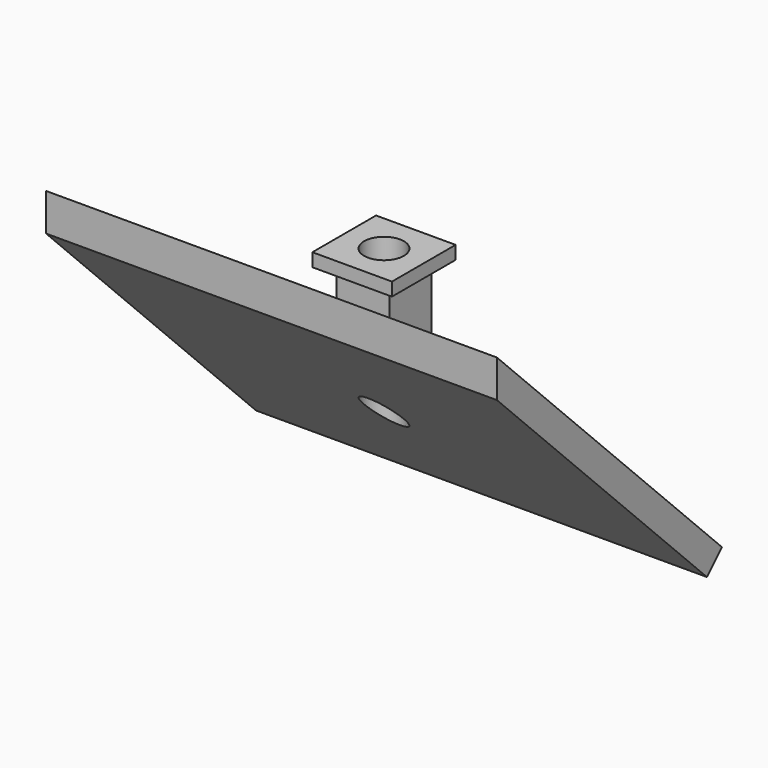
from build123d import *

# Parameters (mm, degrees)
F1_W     = 170
F1_H     = 150
F2_DEPTH = 10
F3_SIZE  = 9.99999
F5_DEPTH = 10
F6_W     = 30
F6_H     = 30
F7_DEPTH = 5
F8_R     = 7.5
F9_DEPTH = 100.1050764009


# Not quite as in the source:
# - a fillet or chamfer is up to 0.001 mm smaller than in the source, because OpenCascade refuses the exact size


with BuildPart() as f2:
    # F1 (on face) → F2 (new body)
    with BuildSketch(Plane(origin=(0, 0, 0), x_dir=(1, 0, 0), z_dir=(0, -0.7071067812, -0.7071067812))):
        Rectangle(F1_W, F1_H)
    extrude(amount=F2_DEPTH)

    # F3 (size 10 in the source; OpenCascade refuses exactly that, so slightly less here)
    f3_edges = [f2.edges().sort_by_distance(p)[0] for p in [
        (0, -60.104076, 45.961941),
    ]]
    chamfer(f3_edges, length=F3_SIZE)

    # F4 (on Right) → F5 (join, symmetric)
    with BuildSketch(Plane.YZ):
        Polygon((-10, 35), (-10, 10), (10, -10), (10, 35), align=None)
    extrude(amount=F5_DEPTH, both=True)

    # F6 (on face) → F7 (join)
    with BuildSketch(Plane.XY.offset(35)):
        Rectangle(F6_W, F6_H)
    extrude(amount=F7_DEPTH)

    # F8 (on face) → F9 (cut, through all)
    with BuildSketch(Plane.XY.offset(40)):
        Circle(F8_R)
    extrude(amount=-F9_DEPTH, mode=Mode.SUBTRACT)


solid = f2.part
